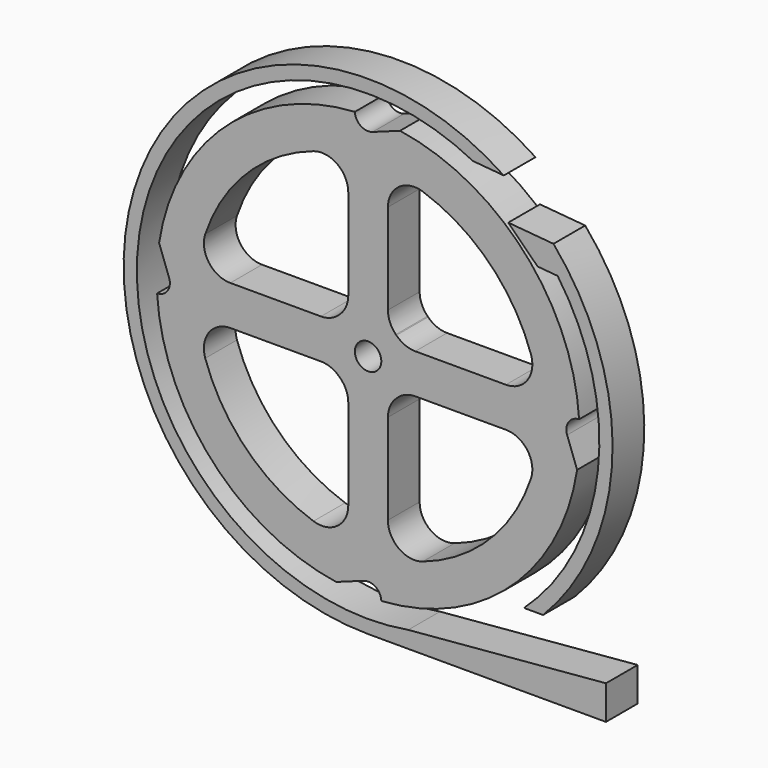
from build123d import *

# Parameters (mm, degrees)
F0_R      = 6.35
F1_DEPTH  = 19.05
F3_DEPTH  = 19.05
F4_R      = 12.7
F5_R      = 117.475
F5_R_2    = 111.125
F6_DEPTH  = 19.05
F8_DEPTH  = 19.05
F9_DEPTH  = 19.05
F11_DEPTH = 19.05
F12_DEPTH = 25.4


with BuildPart() as f1:
    # F0 (on Front) → F1 (new body)
    with BuildSketch(Plane.XZ):
        with BuildLine():
            ThreePointArc((2.1718279101, 95.632951858), (-3.5604804619, 96.3421031885), (-6.3468986567, 101.4015625))
            ThreePointArc((-6.3468986567, 101.4015625), (-68.5661384352, 74.9749602207), (-100.4324652793, 15.3583826596))
            Line((-100.4324652793, 15.3583826596), (-95.632951858, 2.1718279101))
            ThreePointArc((-95.632951858, 2.1718279101), (-96.3421031885, -3.5604804619), (-101.4015625, -6.3468986567))
            ThreePointArc((-101.4015625, -6.3468986567), (-74.9749602207, -68.5661384352), (-15.3583826596, -100.4324652793))
            Line((-15.3583826596, -100.4324652793), (-2.1718279101, -95.632951858))
            ThreePointArc((-2.1718279101, -95.632951858), (3.5604804619, -96.3421031885), (6.3468986567, -101.4015625))
            ThreePointArc((6.3468986567, -101.4015625), (68.5661384352, -74.9749602207), (100.4324652793, -15.3583826596))
            Line((100.4324652793, -15.3583826596), (95.632951858, -2.1718279101))
            ThreePointArc((95.632951858, -2.1718279101), (96.3421031885, 3.5604804619), (101.4015625, 6.3468986567))
            ThreePointArc((101.4015625, 6.3468986567), (74.9749602207, 68.5661384352), (15.3583826596, 100.4324652793))
            Line((15.3583826596, 100.4324652793), (2.1718279101, 95.632951858))
        make_face()
        Circle(F0_R, mode=Mode.SUBTRACT)
    extrude(amount=F1_DEPTH)

    # F2 (on face) → F3 (cut)
    with BuildSketch(Plane.XZ.offset(19.05)):
        with BuildLine():
            ThreePointArc((9.525, 16.4977839421), (13.4703841816, 13.4703841816), (16.4977839421, 9.525))
            Line((16.4977839421, 9.525), (81.9986394704, 9.525))
            ThreePointArc((81.9986394704, 9.525), (58.3716647869, 58.3716647869), (9.525, 81.9986394704))
            Line((9.525, 81.9986394704), (9.525, 16.4977839421))
        make_face()
        with BuildLine():
            ThreePointArc((-16.4977839421, 9.525), (-13.4703841816, 13.4703841816), (-9.525, 16.4977839421))
            Line((-9.525, 16.4977839421), (-9.525, 81.9986394704))
            ThreePointArc((-9.525, 81.9986394704), (-58.3716647869, 58.3716647869), (-81.9986394704, 9.525))
            Line((-81.9986394704, 9.525), (-16.4977839421, 9.525))
        make_face()
        with BuildLine():
            Line((-9.525, -81.9986394704), (-9.525, -16.4977839421))
            ThreePointArc((-9.525, -16.4977839421), (-13.4703841816, -13.4703841816), (-16.4977839421, -9.525))
            Line((-16.4977839421, -9.525), (-81.9986394704, -9.525))
            ThreePointArc((-81.9986394704, -9.525), (-58.3716647869, -58.3716647869), (-9.525, -81.9986394704))
        make_face()
        with BuildLine():
            Line((81.9986394704, -9.525), (16.4977839421, -9.525))
            ThreePointArc((16.4977839421, -9.525), (13.4703841816, -13.4703841816), (9.525, -16.4977839421))
            Line((9.525, -16.4977839421), (9.525, -81.9986394704))
            ThreePointArc((9.525, -81.9986394704), (58.3716647869, -58.3716647869), (81.9986394704, -9.525))
        make_face()
    extrude(amount=-F3_DEPTH, mode=Mode.SUBTRACT)

    # F4
    f4_edges = [f1.edges().sort_by_distance(p)[0] for p in [
        (-9.525, -9.525, 81.998639),
        (-81.998639, -9.525, 9.525),
        (-9.525, -9.525, 16.497784),
        (-16.497784, -9.525, 9.525),
        (81.998639, -9.525, -9.525),
        (9.525, -9.525, 81.998639),
        (9.525, -9.525, 16.497784),
        (16.497784, -9.525, -9.525),
        (16.497784, -9.525, 9.525),
        (81.998639, -9.525, 9.525),
        (9.525, -9.525, -81.998639),
        (9.525, -9.525, -16.497784),
        (-9.525, -9.525, -16.497784),
        (-16.497784, -9.525, -9.525),
        (-81.998639, -9.525, -9.525),
        (-9.525, -9.525, -81.998639),
    ]]
    fillet(f4_edges, radius=F4_R)


with BuildPart() as f6:
    # F5 (on Front) → F6 (new body)
    with BuildSketch(Plane.XZ):
        Circle(F5_R)
        Circle(F5_R_2, mode=Mode.SUBTRACT)
    extrude(amount=F6_DEPTH)

    # F7 (on face) → F8 (join)
    with BuildSketch(Plane.XZ.offset(19.05)):
        with BuildLine():
            ThreePointArc((48.810471892, -106.8546370481), (24.9762601061, -114.7892070541), (0, -117.475))
            Line((0, -117.475), (114.3, -117.475))
            Line((114.3, -117.475), (114.3, -101.125045759))
            Line((114.3, -101.125045759), (48.810471892, -106.8546370481))
        make_face()
    extrude(amount=-F8_DEPTH)

    # F7 (on face) → F9 (cut)
    with BuildSketch(Plane.XZ.offset(19.05)):
        with BuildLine():
            ThreePointArc((74.9163032234, -82.075045759), (49.0528917385, -99.7124838578), (19.2966537432, -109.4367615535))
            Line((19.2966537432, -109.4367615535), (48.810471892, -106.8546370481))
            ThreePointArc((48.810471892, -106.8546370481), (67.5747653841, -96.0938432382), (84.0479773026, -82.075045759))
            Line((84.0479773026, -82.075045759), (74.9163032234, -82.075045759))
        make_face()
    extrude(amount=-F9_DEPTH, mode=Mode.SUBTRACT)

    # F10 (on face) → F11 (join)
    with BuildSketch(Plane.XZ.offset(19.05)):
        Polygon((89.0810143056, 76.582951858), (67.343899207, 78.4847030069), (81.4441892706, 64.5025755371), (91.0838634658, 63.6592133249), align=None)
    extrude(amount=-F11_DEPTH)

    # F10 (on face) → F12 (cut)
    with BuildSketch(Plane.XZ.offset(19.05)):
        Polygon((50.4505131202, 99.0126827781), (64.1809810406, 78.7614224901), (67.343899207, 78.4847030069), (89.0810143056, 76.582951858), (89.0810143056, 95.632951858), align=None)
    extrude(amount=-F12_DEPTH, mode=Mode.SUBTRACT)


solid = Compound([f1.part, f6.part])
